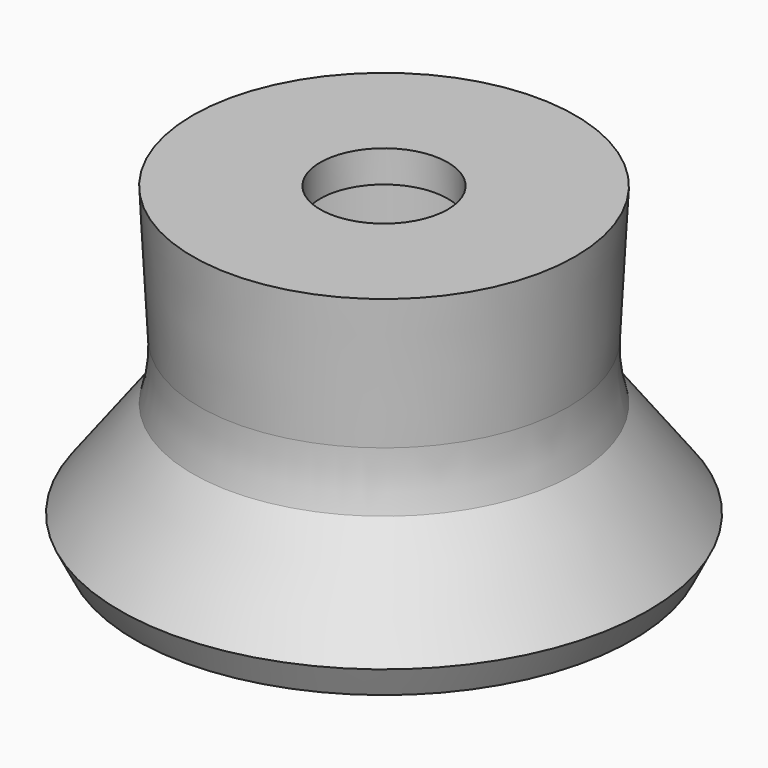
from build123d import *

# Parameters (mm, degrees)
F0_R     = 6
F1_DEPTH = 10
F4_R     = 3.75
F5_DEPTH = 9
F6_R     = 2
F7_DEPTH = 3.5
F11_SIZE = 1.2


# Not quite as in the source:
# - a fillet or chamfer that OpenCascade refuses, or shapes differently, is made with other operations: its cross-section is extruded or revolved along the edge and cut away or added


with BuildPart() as f1:
    # F0 (on Top) → F1 (new body)
    with BuildSketch(Plane.XY):
        Circle(F0_R)
    extrude(amount=F1_DEPTH)

    # F2 (on Right) → F3 (revolve)
    with BuildSketch(Plane.YZ):
        Polygon((9, 0), (6, 4), (6, 0), align=None)
    revolve(axis=Axis((0, 0, 0), (0, 0, 1)))

    # F4 (on face) → F5 (cut)
    with BuildSketch(Plane(origin=(0, 0, 0), x_dir=(1, 0, 0), z_dir=(0, 0, -1))):
        Circle(F4_R)
    extrude(amount=-F5_DEPTH, mode=Mode.SUBTRACT)

    # F6 (on face) → F7 (cut)
    with BuildSketch(Plane(origin=(0, 0, 9), x_dir=(1, 0, 0), z_dir=(0, 0, -1))):
        Circle(F6_R)
    extrude(amount=-F7_DEPTH, mode=Mode.SUBTRACT)

    # F8 (on Front) → F9 (revolve, cut)
    with BuildSketch(Plane.XZ):
        Polygon((6, 4), (6, 10), (5.6855533243, 4), align=None)
    revolve(axis=Axis((0, 0, 10), (0, 0, 1)), mode=Mode.SUBTRACT)

    # F10: fillet of radius 5.08 on 1 edges, made by hand

    # F10_s1 → F10_t2 (revolve)
    with BuildSketch(Plane.XZ):
        with BuildLine():
            ThreePointArc((6, 4), (5.8107107389, 4.8763729429), (5.7784395282, 5.7723743538))
            Line((5.7784395282, 5.7723743538), (5.6769787675, 5.7776916869))
            Line((5.6769787675, 5.7776916869), (5.5840925636, 4.0053173332))
            Line((5.5840925636, 4.0053173332), (5.6855533243, 3.8984))
            ThreePointArc((5.6855533243, 3.8984), (5.8427766622, 3.8984), (5.9029704487, 3.9698698461))
            Line((5.9029704487, 3.9698698461), (6, 4))
        make_face()
    revolve(axis=Axis((0, 0, 4), (0, 0, 1)))

    # F11
    f11_edges = [f1.edges().sort_by_distance(p)[0] for p in [
        (0, -9, 0),
    ]]
    chamfer(f11_edges, length=F11_SIZE)


solid = f1.part
